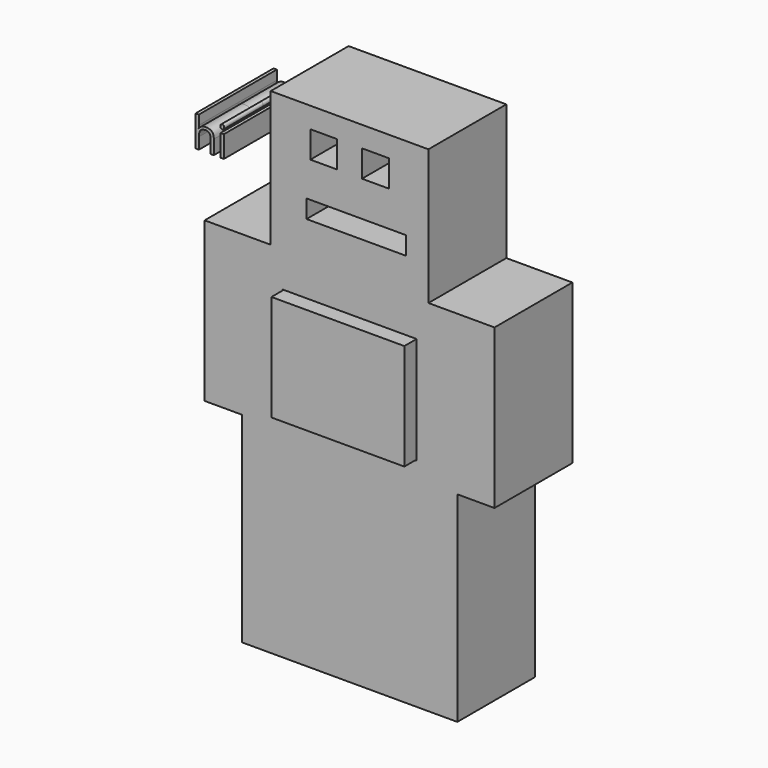
from build123d import *

# Parameters (mm, degrees)
F0_W         = 6.9838857744
F0_H         = 6.9838911295
F0_W_2       = 25.9401509538
F0_H_2       = 4.7390647233
F0_W_3       = 34.9194221199
F0_H_3       = 27.9355458915
F0_TEXT_SIZE = 10.6259870032
F1_DEPTH     = 12.7
F2_W         = 34.6654221199
F2_H         = 27.6815458915
F3_DEPTH     = 16.51


# Not quite as in the source:
# - a feature of the source that left no trace in its solid (it failed there, or was rolled back) is left out
# - Text() gives the source's letters only with a copy of the font that has no kerning and outlines rounded to 1/6400 em; it was checked with that copy


with BuildPart() as f1:
    # F0 (on Front) → F1 (new body, symmetric)
    with BuildSketch(Plane.XZ):
        Polygon((-20.5746181309, 41.4772182703), (0, 41.4772182703), (20.5746181309, 41.4772182703), (20.5746181309, 76.7803711356), (-20.5746181309, 76.7803711356), align=None)
        with Locations((-6.7344576819, 67.8842291236)):
            Rectangle(F0_W, F0_H, mode=Mode.SUBTRACT)
        with Locations((1.7459751107, 52.7940448374)):
            Rectangle(F0_W_2, F0_H_2, mode=Mode.SUBTRACT)
        with Locations((6.7344576819, 67.8842291236)):
            Rectangle(F0_W, F0_H, mode=Mode.SUBTRACT)
        Polygon((20.5746181309, 41.4772182703), (0, 41.4772182703), (-20.5746181309, 41.4772182703), (-37.8166548908, 41.4772182703), (-37.8166548908, 0), (-28.1180106103, 0), (-28.1180106103, -44.7329580784), (0, -44.7329580784), (28.1180106103, -44.7329580784), (28.1180106103, 0), (37.8166548908, 0), (37.8166548908, 41.4772182703), align=None)
        with Locations((0, 18.2487498969)):
            Rectangle(F0_W_3, F0_H_3, mode=Mode.SUBTRACT)
        Polygon((28.1180106103, -52.2763505578), (28.1180106103, -44.7329580784), (0, -44.7329580784), (-28.1180106103, -44.7329580784), (-28.1180106103, -52.2763505578), (0, -52.2763505578), align=None)
        with Locations((-41.0796999931, 57.2127811611)):
            Text('hi', F0_TEXT_SIZE, font='Open Sans', text_align=(TextAlign.LEFT, TextAlign.BOTTOM))
    extrude(amount=F1_DEPTH, both=True)


with BuildPart() as f3:
    # F2 (on Front) → F3 (new body, symmetric)
    with BuildSketch(Plane.XZ):
        with Locations((0, 18.2487498969)):
            Rectangle(F2_W, F2_H)
    extrude(amount=F3_DEPTH, both=True)


solid = Compound([f1.part, f3.part])
